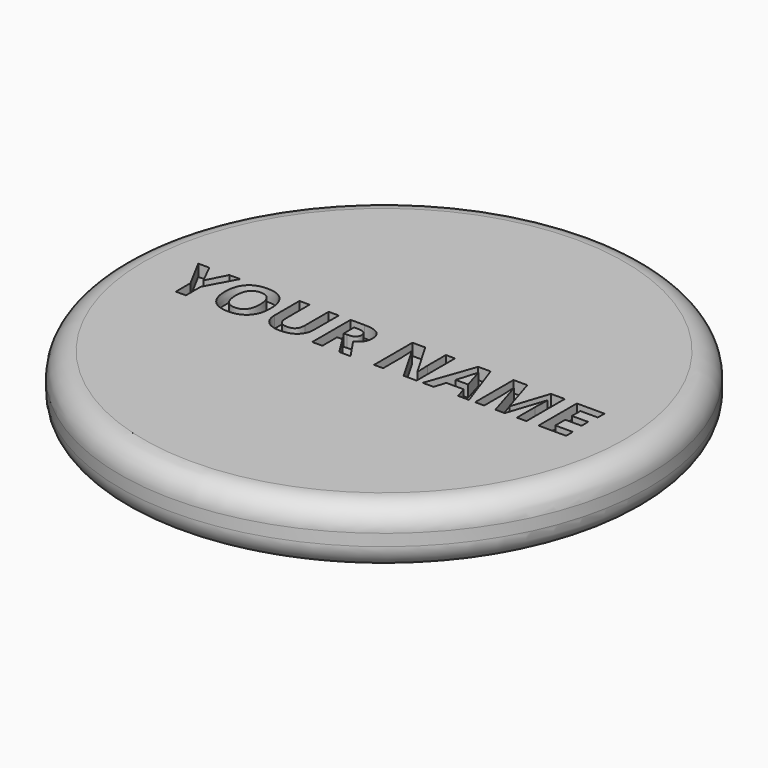
from build123d import *

# Parameters (mm, degrees)
F0_R           = 57.15
F1_DEPTH       = 12.7
F2_R           = 5.08
F3_TEXT_SIZE   = 14.5558739255
F3_TEXT_SIZE_2 = 23.7602923264
F4_DEPTH       = 2.54


# Not quite as in the source:
# - Text() gives the source's letters only with a copy of the font that has no kerning and outlines rounded to 1/6400 em; it was checked with that copy


with BuildPart() as f1:
    # F0 (on Top) → F1 (new body)
    with BuildSketch(Plane.XY):
        Circle(F0_R)
    extrude(amount=F1_DEPTH)

    # F2
    f2_edges = [f1.edges().sort_by_distance(p)[0] for p in [
        (-57.15, 0, 12.7),
        (-57.15, 0, 0),
    ]]
    fillet(f2_edges, radius=F2_R)

    # F3 (on face) → F4 (cut)
    with BuildSketch(Plane.XY.offset(12.7)):
        with Locations((-44.45, -5.1204026494)):
            Text('YOUR NAME', F3_TEXT_SIZE, font='Open Sans', font_style=FontStyle.BOLD, text_align=(TextAlign.LEFT, TextAlign.BOTTOM))
        with Locations((-266.8502926826, -93.7011820519)):
            Text('RUBIN', F3_TEXT_SIZE_2, font='Open Sans', font_style=FontStyle.BOLD, text_align=(TextAlign.LEFT, TextAlign.BOTTOM))
    extrude(amount=-F4_DEPTH, mode=Mode.SUBTRACT)


solid = f1.part
